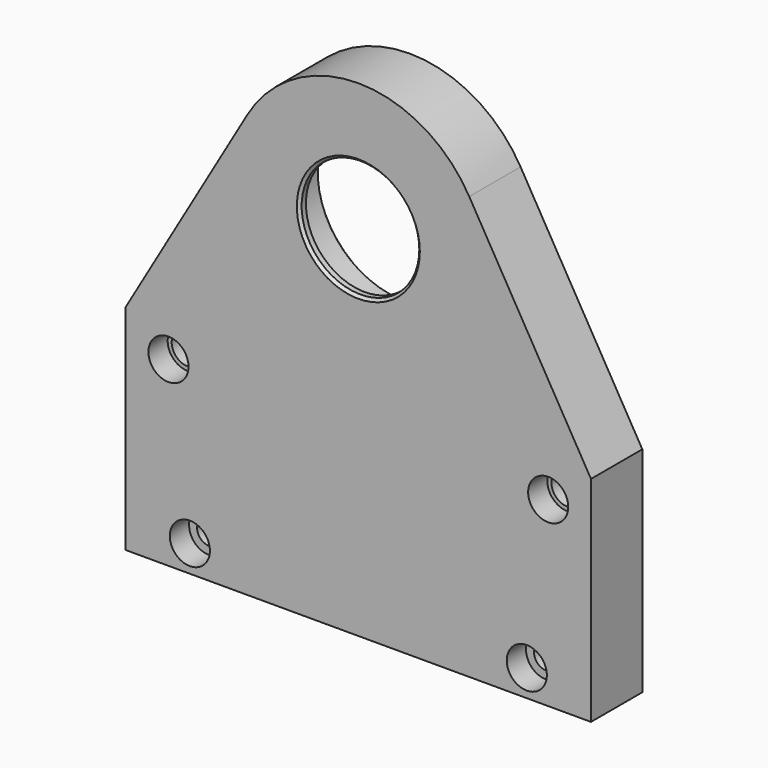
from build123d import *

# Parameters (mm, degrees)
F0_R     = 11
F1_DEPTH = 12
F2_R     = 3
F3_DEPTH = 18
F2_R_2   = 3.75
F4_DEPTH = 4.5
F2_R_3   = 2.25
F5_DEPTH = 12.001
F6_DEPTH = 4.5
F10_SIZE = 0.5


# Not quite as in the source:
# - a pattern or mirror of a feature is missing from the dataset's text; its kind, count and spacing are read off the source's solid


with BuildPart() as f1:
    # F0 (on Front) → F1 (new body)
    with BuildSketch(Plane.XZ):
        with BuildLine():
            Line((-43.5, 40), (-43.5, 0))
            Line((-43.5, 0), (43.5, 0))
            Line((43.5, 0), (43.5, 40))
            Line((43.5, 40), (20.7387457553, 79.0790903836))
            ThreePointArc((20.7387457553, 79.0790903836), (0, 91), (-20.7387457553, 79.0790903836))
            Line((-20.7387457553, 79.0790903836), (-43.5, 40))
        make_face()
        with Locations((0, 67)):
            Circle(F0_R, mode=Mode.SUBTRACT)
    extrude(amount=F1_DEPTH)

    # F2 (on face) → F3 (cut)
    with BuildSketch(Plane.XZ.offset(12)):
        with Locations((-35.5, 34)):
            Circle(F2_R)
    f3 = extrude(amount=-F3_DEPTH, mode=Mode.SUBTRACT)

    # F3_copies: F3 across plane
    add(f3.mirror(Plane(origin=(0, 0, 0), x_dir=(0, 0, 1), z_dir=(1, 0, 0))), mode=Mode.SUBTRACT)

    # F2 (on face) → F4 (cut)
    with BuildSketch(Plane.XZ.offset(12)):
        with Locations((-35.5, 34)):
            Circle(F2_R_2)
        with Locations((-35.5, 34)):
            Circle(F2_R, mode=Mode.SUBTRACT)
    f4 = extrude(amount=-F4_DEPTH, mode=Mode.SUBTRACT)

    # F4_copies: F4 across plane
    add(f4.mirror(Plane(origin=(0, 0, 0), x_dir=(0, 0, 1), z_dir=(1, 0, 0))), mode=Mode.SUBTRACT)

    # F2 (on face) → F5 (cut, through all)
    with BuildSketch(Plane.XZ.offset(12)):
        with Locations((-31.5, 5)):
            Circle(F2_R_3)
    f5 = extrude(amount=-F5_DEPTH, mode=Mode.SUBTRACT)

    # F5_copies: F5 across plane
    add(f5.mirror(Plane(origin=(0, 0, 0), x_dir=(0, 0, 1), z_dir=(1, 0, 0))), mode=Mode.SUBTRACT)

    # F2 (on face) → F6 (cut)
    with BuildSketch(Plane.XZ.offset(12)):
        with Locations((-31.5, 5)):
            Circle(F2_R_2)
        with Locations((-31.5, 5)):
            Circle(F2_R_3, mode=Mode.SUBTRACT)
    f6 = extrude(amount=-F6_DEPTH, mode=Mode.SUBTRACT)

    # F6_copies: F6 across plane
    add(f6.mirror(Plane(origin=(0, 0, 0), x_dir=(0, 0, 1), z_dir=(1, 0, 0))), mode=Mode.SUBTRACT)

    # F8 (on offset) → F9 (revolve, cut)
    with BuildSketch(Plane.XY.offset(67)):
        Polygon((0, 0), (0, -12), (11, -12), (11, -10.5), (13, -10.5), (13, -9), (16, -9), (16, -1.5), (17, -0.5), (20, -0.5), (20, 0), align=None)
    revolve(axis=Axis((0, -9.5826864708, 67), (0, 1, 0)), mode=Mode.SUBTRACT)

    # F10
    f10_edges = [f1.edges().sort_by_distance(p)[0] for p in [
        (-11, -12, 67),
    ]]
    chamfer(f10_edges, length=F10_SIZE)


solid = f1.part
